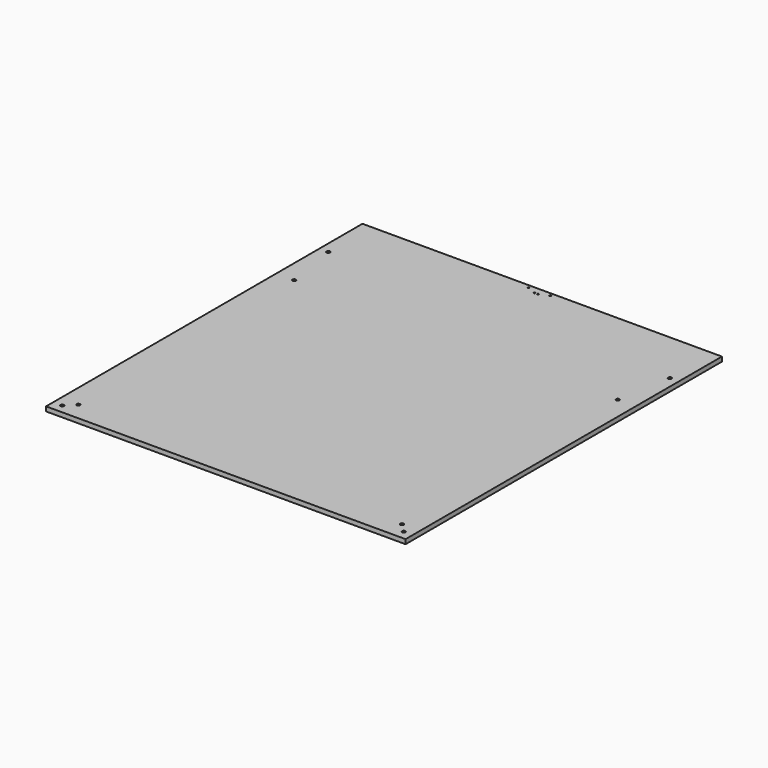
from build123d import *

# Parameters (mm, degrees)
F0_W     = 1016
F0_H     = 1117.6
F1_DEPTH = 12.7
F3_DEPTH = 25.4
F4_R     = 4.7625
F5_DEPTH = 25.4


# Not quite as in the source:
# - a feature names something its author has since deleted; it is built from what else it names


with BuildPart() as f1:
    # F0 (on Top) → F1 (new body)
    with BuildSketch(Plane.XY):
        Rectangle(F0_W, F0_H)
    extrude(amount=F1_DEPTH)

    # F2 (on face) → F3 (cut)
    with BuildSketch(Plane.XY.offset(12.7)):
        with BuildLine():
            Line((-30.559375, 549.275), (-30.559375, 551.65625))
            ThreePointArc((-30.559375, 551.65625), (-32.940625, 549.275), (-30.559375, 546.89375))
            Line((-30.559375, 546.89375), (-30.559375, 549.275))
        make_face()
        with BuildLine():
            ThreePointArc((-28.178125, 549.275), (-28.8755769773, 550.9587980227), (-30.559375, 551.65625))
            Line((-30.559375, 551.65625), (-30.559375, 549.275))
            Line((-30.559375, 549.275), (-28.178125, 549.275))
        make_face()
        with BuildLine():
            Line((-28.178125, 549.275), (-30.559375, 549.275))
            Line((-30.559375, 549.275), (-30.559375, 546.89375))
            ThreePointArc((-30.559375, 546.89375), (-28.8755769773, 547.5912019773), (-28.178125, 549.275))
        make_face()
        with BuildLine():
            Line((-5.159375, 538.1625), (-7.540625, 538.1625))
            ThreePointArc((-7.540625, 538.1625), (-5.159375, 535.78125), (-2.778125, 538.1625))
            Line((-2.778125, 538.1625), (-5.159375, 538.1625))
        make_face()
        with BuildLine():
            ThreePointArc((-2.778125, 538.1625), (-5.159375, 540.54375), (-7.540625, 538.1625))
            Line((-7.540625, 538.1625), (-5.159375, 538.1625))
            Line((-5.159375, 538.1625), (-2.778125, 538.1625))
        make_face()
        with BuildLine():
            Line((5.159375, 538.1625), (7.540625, 538.1625))
            ThreePointArc((7.540625, 538.1625), (5.159375, 540.54375), (2.778125, 538.1625))
            Line((2.778125, 538.1625), (5.159375, 538.1625))
        make_face()
        with BuildLine():
            ThreePointArc((2.778125, 538.1625), (5.159375, 535.78125), (7.540625, 538.1625))
            Line((7.540625, 538.1625), (5.159375, 538.1625))
            Line((5.159375, 538.1625), (2.778125, 538.1625))
        make_face()
        with BuildLine():
            Line((30.559375, 549.275), (30.559375, 551.65625))
            ThreePointArc((30.559375, 551.65625), (28.8755769773, 550.9587980227), (28.178125, 549.275))
            Line((28.178125, 549.275), (30.559375, 549.275))
        make_face()
        with BuildLine():
            Line((30.559375, 546.89375), (30.559375, 549.275))
            Line((30.559375, 549.275), (28.178125, 549.275))
            ThreePointArc((28.178125, 549.275), (28.8755769773, 547.5912019773), (30.559375, 546.89375))
        make_face()
        with BuildLine():
            ThreePointArc((32.940625, 549.275), (32.2431730227, 550.9587980227), (30.559375, 551.65625))
            Line((30.559375, 551.65625), (30.559375, 549.275))
            Line((30.559375, 549.275), (30.559375, 546.89375))
            ThreePointArc((30.559375, 546.89375), (32.2431730227, 547.5912019773), (32.940625, 549.275))
        make_face()
    extrude(amount=-F3_DEPTH, mode=Mode.SUBTRACT)

    # F4 (on face) → F5 (cut)
    with BuildSketch(Plane.XY.offset(12.7)):
        with Locations((-482.6, 406.4)):
            Circle(F4_R)
        with BuildLine():
            Line((-457.2, 254), (-461.9625, 254))
            ThreePointArc((-461.9625, 254), (-457.2, 249.2375), (-452.4375, 254))
            ThreePointArc((-452.4375, 254), (-453.8324039546, 257.3675960454), (-457.2, 258.7625))
            Line((-457.2, 258.7625), (-457.2, 254))
        make_face()
        with BuildLine():
            ThreePointArc((-457.2, 258.7625), (-460.5675960454, 257.3675960454), (-461.9625, 254))
            Line((-461.9625, 254), (-457.2, 254))
            Line((-457.2, 254), (-457.2, 258.7625))
        make_face()
        with Locations((-482.6, -533.4)):
            Circle(F4_R)
        with BuildLine():
            Line((-457.2, -508), (-457.2, -512.7625))
            ThreePointArc((-457.2, -512.7625), (-453.8324039546, -511.3675960454), (-452.4375, -508))
            ThreePointArc((-452.4375, -508), (-457.2, -503.2375), (-461.9625, -508))
            Line((-461.9625, -508), (-457.2, -508))
        make_face()
        with BuildLine():
            ThreePointArc((-461.9625, -508), (-460.5675960454, -511.3675960454), (-457.2, -512.7625))
            Line((-457.2, -512.7625), (-457.2, -508))
            Line((-457.2, -508), (-461.9625, -508))
        make_face()
        with Locations((482.6, -533.4)):
            Circle(F4_R)
        with BuildLine():
            Line((457.2, -508), (457.2, -512.7625))
            ThreePointArc((457.2, -512.7625), (460.5675960454, -511.3675960454), (461.9625, -508))
            Line((461.9625, -508), (457.2, -508))
        make_face()
        with BuildLine():
            ThreePointArc((461.9625, -508), (453.8324039546, -504.6324039546), (457.2, -512.7625))
            Line((457.2, -512.7625), (457.2, -508))
            Line((457.2, -508), (461.9625, -508))
        make_face()
        with BuildLine():
            ThreePointArc((457.2, 258.7625), (453.8324039546, 250.6324039546), (461.9625, 254))
            Line((461.9625, 254), (457.2, 254))
            Line((457.2, 254), (457.2, 258.7625))
        make_face()
        with BuildLine():
            Line((457.2, 254), (461.9625, 254))
            ThreePointArc((461.9625, 254), (460.5675960454, 257.3675960454), (457.2, 258.7625))
            Line((457.2, 258.7625), (457.2, 254))
        make_face()
        with Locations((482.6, 406.4)):
            Circle(F4_R)
    extrude(amount=-F5_DEPTH, mode=Mode.SUBTRACT)


solid = f1.part
